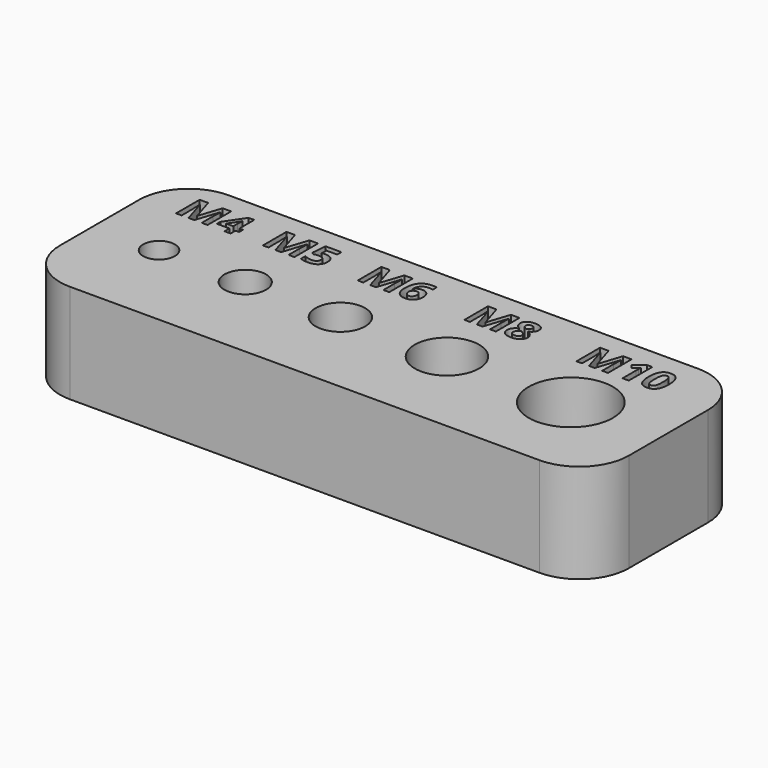
from build123d import *

# Parameters (mm, degrees)
F0_W         = 57.4
F0_H         = 20
F0_R         = 1.6
F0_R_2       = 2.1
F0_R_3       = 2.5
F0_R_4       = 3.25
F0_R_5       = 4.25
F1_DEPTH     = 10
F2_TEXT_SIZE = 4.1666666667
F3_DEPTH     = 1
F4_R         = 5


# Not quite as in the source:
# - Text() gives the source's letters only with a copy of the font that has no kerning and outlines rounded to 1/6400 em; it was checked with that copy


with BuildPart() as f1:
    # F0 (on Top) → F1 (new body)
    with BuildSketch(Plane.XY):
        with Locations((3.8, 0.75)):
            Rectangle(F0_W, F0_H)
        with Locations((-18.3, 0)):
            Circle(F0_R, mode=Mode.SUBTRACT)
        with Locations((-9.6, 0)):
            Circle(F0_R_2, mode=Mode.SUBTRACT)
        Circle(F0_R_3, mode=Mode.SUBTRACT)
        with Locations((10.75, 0)):
            Circle(F0_R_4, mode=Mode.SUBTRACT)
        with Locations((23.25, 0)):
            Circle(F0_R_5, mode=Mode.SUBTRACT)
    extrude(amount=F1_DEPTH)

    # F2 (on face) → F3 (cut)
    with BuildSketch(Plane.XY.offset(10)):
        with Locations((-21.555859375, 5.75)):
            Text('M4', F2_TEXT_SIZE, font='Open Sans', font_style=FontStyle.BOLD, text_align=(TextAlign.LEFT, TextAlign.BOTTOM))
        with Locations((-12.7949869792, 5.75)):
            Text('M5', F2_TEXT_SIZE, font='Open Sans', font_style=FontStyle.BOLD, text_align=(TextAlign.LEFT, TextAlign.BOTTOM))
        with Locations((-3.2223307292, 5.75)):
            Text('M6', F2_TEXT_SIZE, font='Open Sans', font_style=FontStyle.BOLD, text_align=(TextAlign.LEFT, TextAlign.BOTTOM))
        with Locations((7.5338541667, 5.75)):
            Text('M8', F2_TEXT_SIZE, font='Open Sans', font_style=FontStyle.BOLD, text_align=(TextAlign.LEFT, TextAlign.BOTTOM))
        with Locations((18.8466796875, 5.75)):
            Text('M10', F2_TEXT_SIZE, font='Open Sans', font_style=FontStyle.BOLD, text_align=(TextAlign.LEFT, TextAlign.BOTTOM))
    extrude(amount=-F3_DEPTH, mode=Mode.SUBTRACT)

    # F4
    f4_edges = [f1.edges().sort_by_distance(p)[0] for p in [
        (32.5, -9.25, 5),
        (32.5, 10.75, 5),
        (-24.9, 10.75, 5),
        (-24.9, -9.25, 5),
    ]]
    fillet(f4_edges, radius=F4_R)


solid = f1.part
